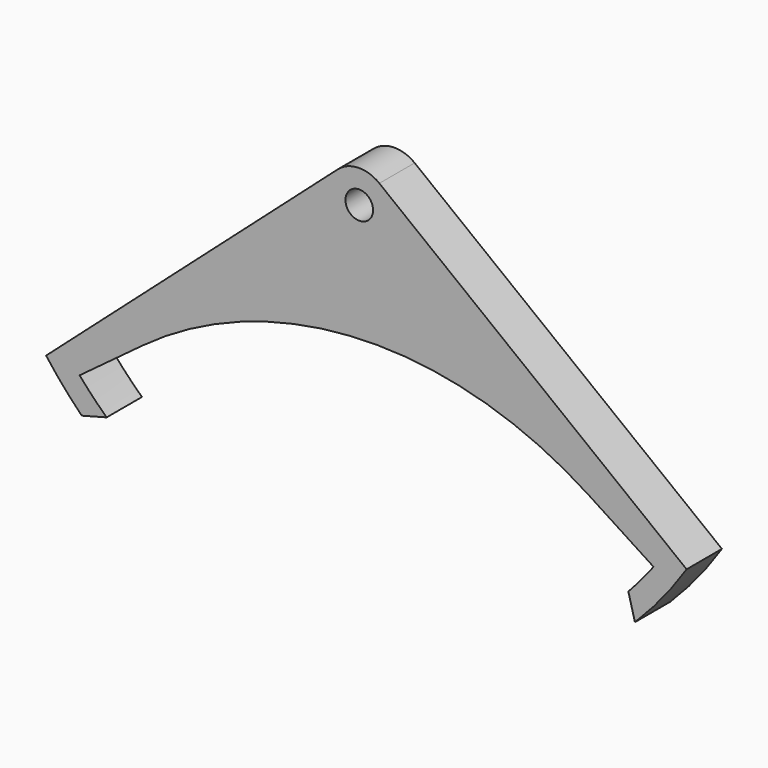
from build123d import *

# Parameters (mm, degrees)
F1_DEPTH = 8
F2_R     = 2.5
F3_DEPTH = 8


# Not quite as in the source:
# - ends of sketch curves that miss each other by under 0.0002 mm in the source are joined


with BuildPart() as f1:
    # F0 (on Front) → F1 (new body)
    with BuildSketch(Plane.XZ):
        with BuildLine():
            ThreePointArc((-58.0214256358, -20.2643207275), (-54.9218439489, -24.1190997792), (-51.5609168942, -27.7482728949))
            Line((-51.5609168942, -27.7482728949), (-47.048692, -26.555894))
            ThreePointArc((-47.048692, -26.555894), (-49.5674409521, -24.0619501846), (-51.9504921504, -21.4380372685))
            Line((-51.9504921504, -21.4380372685), (-40.598231, -13.017462))
            ThreePointArc((-40.598231, -13.017462), (-0.6084110144, 0.8961956506), (40.1770750491, -10.4756859243))
            Line((40.1770750491, -10.4756859243), (52.036298, -18.165861))
            ThreePointArc((52.036298, -18.165861), (49.8229328445, -20.9344101577), (47.4659668709, -23.5817788788))
            Line((47.4659668709, -23.5817788788), (48.658346, -28.094004))
            ThreePointArc((48.658346, -28.094004), (53.6407391456, -22.5987377774), (58.0214266089, -16.6127733984))
            Line((58.0214266089, -16.6127733984), (2.355576, 26.843505))
            ThreePointArc((2.355576, 26.843505), (-1.4641584631, 28.091083381), (-5.1978982267, 26.6058182555))
            Line((-5.1978982267, 26.6058182555), (-58.0214256358, -20.2643207275))
        make_face()
    extrude(amount=F1_DEPTH)

    # F2 (on face) → F3 (cut, through all)
    with BuildSketch(Plane.XZ.offset(8)):
        with Locations((-1.27842, 22.188493)):
            Circle(F2_R)
    extrude(amount=-F3_DEPTH, mode=Mode.SUBTRACT)


solid = f1.part
